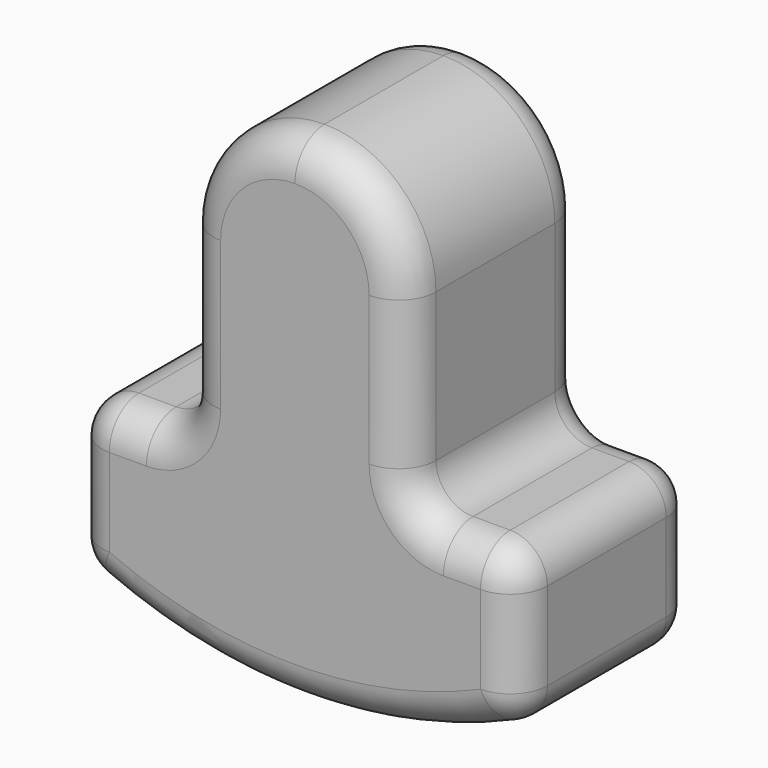
from build123d import *

# Parameters (mm, degrees)
F1_DEPTH = 30
F2_R     = 29.99999
F3_R     = 10


# Not quite as in the source:
# - a fillet or chamfer is up to 0.001 mm smaller than in the source, because OpenCascade refuses the exact size


with BuildPart() as f1:
    # F0 (on Front) → F1 (new body, symmetric)
    with BuildSketch(Plane.XZ):
        with BuildLine():
            Line((30, -5), (30, 75))
            Line((30, 75), (-30, 75))
            Line((-30, 75), (-30, -5))
            Line((-30, -5), (-60, -5))
            Line((-60, -5), (-60, -45))
            ThreePointArc((-60, -45), (0, -59.0661337755), (60, -45))
            Line((60, -45), (60, -5))
            Line((60, -5), (30, -5))
        make_face()
    extrude(amount=F1_DEPTH, both=True)

    # F2 (radius 30 in the source; OpenCascade refuses exactly that, so slightly less here)
    f2_edges = [f1.edges().sort_by_distance(p)[0] for p in [
        (30, 0, 75),
        (-30, 0, 75),
    ]]
    fillet(f2_edges, radius=F2_R)

    # F3
    f3_edges = [f1.edges().sort_by_distance(p)[0] for p in [
        (30, -30, 20.000005),
        (21.213206, -30, 66.213206),
        (45, -30, -5),
        (0, -30, 75),
        (60, -30, -25),
        (-21.213206, -30, 66.213206),
        (0, -30, -59.066134),
        (-30, -30, 20.000005),
        (-60, -30, -25),
        (-45, -30, -5),
        (30, 30, 20.000005),
        (30, 0, 45.00001),
        (30, 0, -5),
        (60, 30, -25),
        (60, 0, -5),
        (60, 0, -45),
        (-30, 0, -5),
        (-45, 30, -5),
        (-60, 0, -5),
        (21.213206, 30, 66.213206),
        (45, 30, -5),
        (0, 30, 75),
        (-21.213206, 30, 66.213206),
        (0, 30, -59.066134),
        (-30, 30, 20.000005),
        (-60, 30, -25),
        (-60, 0, -45),
    ]]
    fillet(f3_edges, radius=F3_R)


solid = f1.part
